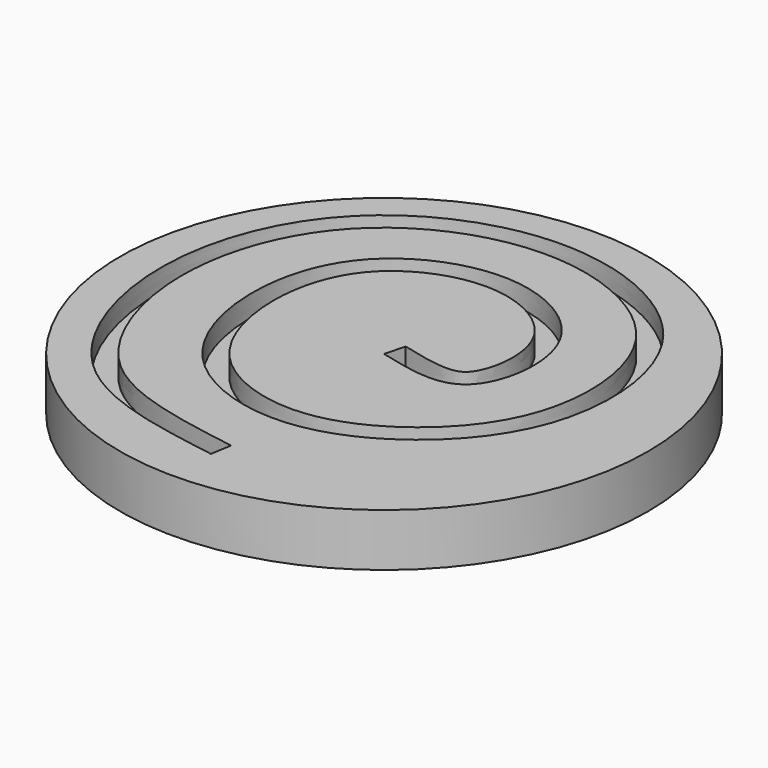
from build123d import *

# Parameters (mm, degrees)
F0_R     = 50
F1_DEPTH = 10
F3_DEPTH = 4


# Not quite as in the source:
# - the dataset's text gives a spline's control points without its knots; the knots are read off the source's solid


with BuildPart() as f1:
    # F0 (on Top) → F1 (new body)
    with BuildSketch(Plane.XY):
        Circle(F0_R)
    extrude(amount=F1_DEPTH)

    # F2 (on face) → F3 (cut)
    with BuildSketch(Plane.XY.offset(10)):
        with BuildLine():
            Line((0.9829752457, 3.8773392509), (0, 0))
            add(Edge.make_bspline(
                [(0, 0), (6.1989170972, -1.5715369903), (18.3009054469, -4.5820748684), (22.2708690558, 21.098136745), (0.0735061662, 34.2606933049), (-24.696823294, 23.9432686999), (-29.5777293656, -0.2026812836), (-21.242860416, -21.0513155032), (0.3063219845, -28.9137402116), (20.8650084968, -20.9802440135), (37.2875332391, -1.1549707016), (34.1376870072, 33.13508074), (-0.1754280995, 48.8840289104), (-35.2364717279, 34.8889421314), (-47.3259993463, 0.3519769186), (-33.9018786494, -35.4686194222), (-11.7437604148, -39.0679776254), (0, -40.9867800772)],
                knots=[0, 0, 0, 0, 0.0525535116, 0.1096237828, 0.1717910753, 0.2358694433, 0.2986406084, 0.3592346609, 0.4192497264, 0.4797384354, 0.5450690227, 0.6175302469, 0.6936624619, 0.7710104122, 0.8480266768, 0.9244411097, 1, 1, 1, 1], degree=3))
            Line((0, -40.9867800772), (0.6450036004, -37.0391262986))
            add(Edge.make_bspline(
                [(0.9829752457, 3.8773392509), (1.9028873637, 3.6441249816), (3.6919433345, 3.1919843928), (5.7605675211, 2.732785135), (7.2810865736, 2.4662486899), (8.3436670607, 2.3240819174), (9.3169618233, 2.2451010951), (10.1887915864, 2.2314853541), (10.947954819, 2.2809860032), (11.5874524899, 2.3861900884), (12.0224756906, 2.5106115901), (12.3206036207, 2.6274021611), (12.5231974111, 2.7234627921), (12.709265499, 2.8287745147), (12.8547684896, 2.9260651259), (12.9537303385, 3.0007327444), (13.0097922913, 3.045623949), (13.065405617, 3.0919209765), (13.1368063649, 3.1548250553), (13.2546992489, 3.2666505482), (13.4080975553, 3.4280372783), (13.5988320235, 3.6574645444), (13.793011554, 3.9228491254), (14.0523488215, 4.3238331909), (14.3698276971, 4.9106602674), (14.7198907044, 5.7375729872), (15.0236752247, 6.6693304102), (15.2697160876, 7.686882739), (15.4495979877, 8.7708840237), (15.5572225131, 9.902137312), (15.5883189477, 11.0617303408), (15.5401508393, 12.231076471), (15.4113885134, 13.3919517708), (15.2369603106, 14.3374724452), (15.0579074215, 15.0722309945), (14.9042054761, 15.6104471009), (14.760291964, 16.0466031193), (14.6359044176, 16.3872240146), (14.5380910297, 16.6382401352), (14.4356903614, 16.8849254649), (14.2918948991, 17.210992659), (14.0990774833, 17.6122224287), (13.8469224085, 18.0839965323), (13.4834359088, 18.7000121361), (12.9785967796, 19.4455949123), (12.2945069159, 20.2998886289), (11.5351348638, 21.1114625837), (10.4272090237, 22.132602539), (8.873962516, 23.2862338072), (6.78302844, 24.4452320191), (4.8933370416, 25.200524048), (3.3207203095, 25.6669467244), (2.1179315126, 25.9454931128), (1.1022148065, 26.1164417869), (0.2849894908, 26.215627576), (-0.3288668952, 26.2710020117), (-0.944832867, 26.3073524442), (-1.7702133334, 26.3307890904), (-2.8071733381, 26.313405725), (-4.0551806217, 26.21906102), (-5.7169415053, 25.9971300145), (-7.776464249, 25.5433043019), (-10.175118105, 24.7317187281), (-12.4562742148, 23.6720925147), (-14.2229522716, 22.6009268113), (-15.5351787337, 21.6437533778), (-16.4640394874, 20.8791496162), (-17.1882331249, 20.2059180499), (-17.7356138092, 19.6474264532), (-18.0639925936, 19.2904481563), (-18.3182625473, 19.0002846122), (-18.5667183142, 18.7072694742), (-18.8683379851, 18.3334029952), (-19.2160160161, 17.8729710371), (-19.6608298312, 17.2435341442), (-20.1819960766, 16.4281771031), (-20.7523934885, 15.4060137367), (-21.268217967, 14.3424853647), (-21.8835524824, 12.87300129), (-22.5172852058, 10.947363596), (-23.0623530621, 8.5233456031), (-23.3946478659, 6.0188215741), (-23.4981201142, 3.8938329372), (-23.4802667425, 2.1893181877), (-23.4176091372, 0.9133395254), (-23.3069435996, -0.3556891252), (-23.1493340787, -1.6091936827), (-22.9448171574, -2.8450597271), (-22.6100002441, -4.4652743304), (-22.0757554184, -6.4318515305), (-21.25283637, -8.6762072748), (-20.4189605639, -10.4336444958), (-19.6650960756, -11.7631346357), (-19.0567723277, -12.720130822), (-18.4059032739, -13.6352485857), (-17.7126959927, -14.5069630382), (-17.0998540199, -15.1960044902), (-16.5882045354, -15.7243596211), (-16.1941571325, -16.1086306674), (-15.7879294574, -16.4824981344), (-15.2290443776, -16.9682925043), (-14.4997105828, -17.5505796161), (-13.5783323537, -18.2079519881), (-12.2929772431, -19.0269758129), (-10.5888047789, -19.938837613), (-8.4196382692, -20.8414361792), (-6.1604276162, -21.5414857343), (-4.2323299068, -21.9485938568), (-2.6807417172, -22.1651690422), (-1.5171397493, -22.2724472773), (-0.5511123318, -22.3154922103), (0.2167258913, -22.3219449036), (0.9831444969, -22.309789572), (1.9389300412, -22.2600968514), (3.4632384995, -22.1083304633), (5.3591482036, -21.7854976699), (7.6163004907, -21.1919650386), (9.8505364688, -20.3990053996), (12.0551163104, -19.4138057378), (13.8608742765, -18.4392396328), (15.2822022906, -17.5719125708), (16.159908179, -16.9942832498), (16.8550219419, -16.5115327951), (17.5455608481, -16.0150277494), (18.3959762693, -15.3715302931), (19.3933777801, -14.5631467928), (20.6890981922, -13.4376059632), (22.238475441, -11.9422761323), (23.9662259333, -10.0095081517), (25.5445342883, -7.9408680127), (26.956502869, -5.7378373633), (27.9811372935, -3.7900027382), (28.7017933347, -2.1635587764), (29.1907558737, -0.909201038), (29.6262446766, 0.3803481443), (30.0058614184, 1.7053748031), (30.3298836132, 3.0721528042), (30.6850577494, 4.9406805374), (30.9807318974, 7.3489690424), (31.0870049589, 10.3078079807), (30.9362916645, 13.2888755712), (30.5225277046, 16.2461741816), (29.9553697607, 18.6534779374), (29.3674099953, 20.5237371037), (28.859293606, 21.8936146039), (28.2840401957, 23.2258374812), (27.6416920127, 24.5158570639), (27.0505011679, 25.5521651048), (26.5439476352, 26.3560493273), (26.2133379148, 26.8476041708), (25.9403841004, 27.2341423925), (25.6609301543, 27.6174320909), (25.2998089096, 28.0900254247), (24.8478148423, 28.6466754627), (24.2207795279, 29.3746517677), (23.3921466434, 30.2575058744), (22.3290787981, 31.2718684755), (21.200584435, 32.2393418762), (19.6134002178, 33.4642423036), (17.483944727, 34.8684997774), (14.7279424465, 36.335261054), (11.8057697751, 37.5692599456), (8.7534005683, 38.5574407969), (6.1320587685, 39.1664353827), (4.0070592021, 39.5199677194), (2.4041134062, 39.7171950002), (0.7963798197, 39.845544794), (-0.8104146587, 39.9039396847), (-2.4185221304, 39.8924871177), (-4.5604842374, 39.7855984688), (-7.2265028263, 39.4825428059), (-10.383273289, 38.8561669397), (-13.4730023265, 37.9761953251), (-16.4709730035, 36.8525213366), (-19.3525929616, 35.495793691), (-22.0936516014, 33.9173549474), (-24.2410679288, 32.4271611991), (-25.8655925512, 31.1362572648), (-27.0345467632, 30.1202513865), (-28.1514618479, 29.0579692759), (-29.2135354163, 27.9508796299), (-30.2247884904, 26.7954443816), (-31.5040107866, 25.1941068986), (-32.9728421502, 23.0827380752), (-34.5230333925, 20.3897950674), (-35.8563298141, 17.5545162934), (-36.9680228455, 14.5947878667), (-37.8534777088, 11.5292202804), (-38.50829185, 8.37697423), (-38.9284090709, 5.1576759205), (-39.0798568641, 2.4353735099), (-39.0802229594, 0.2441356766), (-39.019674873, -1.404526295), (-38.8987000057, -3.0556956999), (-38.6576677887, -5.2535089233), (-38.208530677, -7.9821164763), (-37.4395364197, -11.1883361085), (-36.448526432, -14.2886044617), (-35.2450434282, -17.2455446794), (-33.8403020237, -20.0226537749), (-32.2472533044, -22.5849192117), (-30.7749066354, -24.5139138673), (-29.6749561406, -25.7433689609), (-29.0275267795, -26.4098685759), (-28.5327604029, -26.8913330618), (-28.1128643996, -27.2770255237), (-27.7727202041, -27.5758956289), (-27.2564166682, -28.0161642198), (-26.4588116506, -28.6472818821), (-25.3448536883, -29.4309811538), (-24.1795231027, -30.160947193), (-22.962356162, -30.840670048), (-21.2704230555, -31.6840980598), (-19.0271487492, -32.6276377811), (-16.139427244, -33.6044672294), (-13.0711447396, -34.448651841), (-9.8404866183, -35.1853006191), (-5.342352494, -36.061021054), (-1.7839882341, -36.6422555074), (0.6450036004, -37.0391262986)],
                knots=[0, 0, 0, 0, 0.0078125, 0.015625, 0.01953125, 0.0234375, 0.02734375, 0.03125, 0.03515625, 0.0390625, 0.04296875, 0.044921875, 0.046875, 0.048828125, 0.05078125, 0.0517578125, 0.0522460938, 0.052734375, 0.0537109375, 0.0546875, 0.056640625, 0.05859375, 0.060546875, 0.0625, 0.06640625, 0.0703125, 0.07421875, 0.078125, 0.08203125, 0.0859375, 0.08984375, 0.09375, 0.09765625, 0.1015625, 0.103515625, 0.10546875, 0.107421875, 0.1083984375, 0.109375, 0.1103515625, 0.111328125, 0.11328125, 0.115234375, 0.1171875, 0.12109375, 0.125, 0.12890625, 0.1328125, 0.140625, 0.1484375, 0.15625, 0.16015625, 0.1640625, 0.16796875, 0.169921875, 0.171875, 0.173828125, 0.17578125, 0.1796875, 0.18359375, 0.1875, 0.1953125, 0.203125, 0.2109375, 0.21875, 0.22265625, 0.2265625, 0.23046875, 0.232421875, 0.234375, 0.2353515625, 0.236328125, 0.23828125, 0.240234375, 0.2421875, 0.24609375, 0.25, 0.25390625, 0.2578125, 0.265625, 0.2734375, 0.28125, 0.2890625, 0.29296875, 0.296875, 0.30078125, 0.3046875, 0.30859375, 0.3125, 0.3203125, 0.328125, 0.3359375, 0.33984375, 0.34375, 0.34765625, 0.3515625, 0.35546875, 0.357421875, 0.359375, 0.361328125, 0.36328125, 0.3671875, 0.37109375, 0.375, 0.3828125, 0.390625, 0.3984375, 0.40625, 0.41015625, 0.4140625, 0.41796875, 0.419921875, 0.421875, 0.42578125, 0.4296875, 0.4375, 0.4453125, 0.453125, 0.4609375, 0.46875, 0.47265625, 0.4765625, 0.478515625, 0.48046875, 0.484375, 0.48828125, 0.4921875, 0.5, 0.5078125, 0.515625, 0.5234375, 0.53125, 0.53515625, 0.5390625, 0.54296875, 0.546875, 0.55078125, 0.5546875, 0.5625, 0.5703125, 0.578125, 0.5859375, 0.59375, 0.59765625, 0.6015625, 0.60546875, 0.609375, 0.61328125, 0.615234375, 0.6171875, 0.6181640625, 0.619140625, 0.62109375, 0.623046875, 0.625, 0.62890625, 0.6328125, 0.63671875, 0.640625, 0.6484375, 0.65625, 0.6640625, 0.671875, 0.6796875, 0.68359375, 0.6875, 0.69140625, 0.6953125, 0.69921875, 0.703125, 0.7109375, 0.71875, 0.7265625, 0.734375, 0.7421875, 0.75, 0.7578125, 0.76171875, 0.765625, 0.76953125, 0.7734375, 0.77734375, 0.78125, 0.7890625, 0.796875, 0.8046875, 0.8125, 0.8203125, 0.828125, 0.8359375, 0.84375, 0.84765625, 0.8515625, 0.85546875, 0.859375, 0.8671875, 0.875, 0.8828125, 0.890625, 0.8984375, 0.90625, 0.9140625, 0.91796875, 0.919921875, 0.921875, 0.923828125, 0.9248046875, 0.92578125, 0.9296875, 0.93359375, 0.9375, 0.94140625, 0.9453125, 0.953125, 0.9609375, 0.96875, 0.9765625, 0.984375, 1, 1, 1, 1], degree=3))
        make_face()
    extrude(amount=-F3_DEPTH, mode=Mode.SUBTRACT)


solid = f1.part
